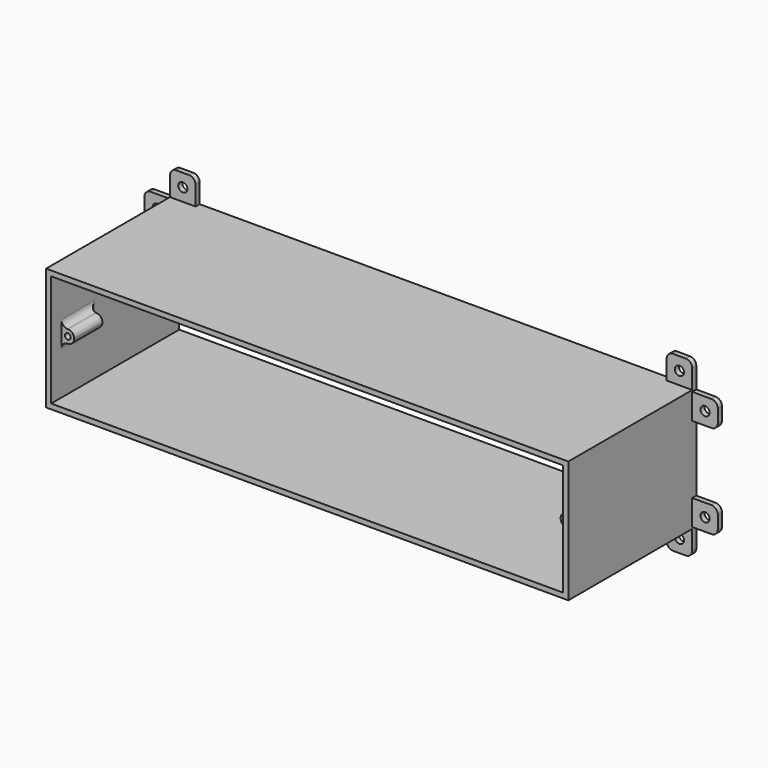
from build123d import *

# Parameters (mm, degrees)
F1_DEPTH     = 50
F0_W         = 8
F0_H         = 8
F0_R         = 1.425
F2_DEPTH     = 1.6
F3_R         = 2
F5_R         = 2
F6_START     = 35
F0_W_2       = 4
F0_H_2       = 4
F0_R_2       = 0.9
F6_DEPTH     = 11
F7_T1_DEPTH  = 11
F7_T6_DEPTH  = 4
F7_S7_R      = 0.9
F7_T8_DEPTH  = 4
F7_T13_DEPTH = 9
F7_T17_DEPTH = 16
F7_T24_DEPTH = 9
F7_T28_DEPTH = 16
F7_T31_DEPTH = 21
F9_R         = 2


# Not quite as in the source:
# - a fillet or chamfer that OpenCascade refuses, or shapes differently, is made with other operations: its cross-section is extruded or revolved along the edge and cut away or added


with BuildPart() as f1:
    # F0 (on Front) → F1 (new body)
    with BuildSketch(Plane.XZ):
        Polygon((-81.6, -18.6015841149), (-81.6, -19.1), (-73.6, -19.1), (73.6, -19.1), (81.6, -19.1), (81.6, -18.6015841149), (81.6, -10.6015841149), (81.6, 10.6015841149), (81.6, 18.6015841149), (81.6, 19.1), (73.6, 19.1), (-73.6, 19.1), (-81.6, 19.1), (-81.6, 18.6015841149), (-81.6, 10.6015841149), (-81.6, -10.6015841149), align=None)
        Polygon((80, -2), (80, -17.5), (-80, -17.5), (-80, 17.5), (80, 17.5), (80, 2), align=None, mode=Mode.SUBTRACT)
    extrude(amount=F1_DEPTH)

    # F0 (on Front) → F2 (join)
    with BuildSketch(Plane.XZ):
        Polygon((-81.6, -18.6015841149), (-81.6, -19.1), (-73.6, -19.1), (73.6, -19.1), (81.6, -19.1), (81.6, -18.6015841149), (81.6, -10.6015841149), (81.6, 10.6015841149), (81.6, 18.6015841149), (81.6, 19.1), (73.6, 19.1), (-73.6, 19.1), (-81.6, 19.1), (-81.6, 18.6015841149), (-81.6, 10.6015841149), (-81.6, -10.6015841149), align=None)
        Polygon((80, -2), (80, -17.5), (-80, -17.5), (-80, 17.5), (80, 17.5), (80, 2), align=None, mode=Mode.SUBTRACT)
        with Locations((-77.6, -23.1)):
            Rectangle(F0_W, F0_H)
        with Locations((-77.6, -23.1)):
            Circle(F0_R, mode=Mode.SUBTRACT)
        with Locations((-85.6, -14.6015841149)):
            Rectangle(F0_W, F0_H)
        with Locations((-85.6, -14.6015841149)):
            Circle(F0_R, mode=Mode.SUBTRACT)
        with Locations((77.6, -23.1)):
            Rectangle(F0_W, F0_H)
        with Locations((77.6, -23.1)):
            Circle(F0_R, mode=Mode.SUBTRACT)
        with Locations((-85.6, 14.6015841149)):
            Rectangle(F0_W, F0_H)
        with Locations((-85.6, 14.6015841149)):
            Circle(F0_R, mode=Mode.SUBTRACT)
        with Locations((85.6, -14.6015841149)):
            Rectangle(F0_W, F0_H)
        with Locations((85.6, -14.6015841149)):
            Circle(F0_R, mode=Mode.SUBTRACT)
        with Locations((-77.6, 23.1)):
            Rectangle(F0_W, F0_H)
        with Locations((-77.6, 23.1)):
            Circle(F0_R, mode=Mode.SUBTRACT)
        with Locations((85.6, 14.6015841149)):
            Rectangle(F0_W, F0_H)
        with Locations((85.6, 14.6015841149)):
            Circle(F0_R, mode=Mode.SUBTRACT)
        with Locations((77.6, 23.1)):
            Rectangle(F0_W, F0_H)
        with Locations((77.6, 23.1)):
            Circle(F0_R, mode=Mode.SUBTRACT)
    extrude(amount=F2_DEPTH)

    # F3
    f3_edges = [f1.edges().sort_by_distance(p)[0] for p in [
        (-81.6, -0.8, 27.1),
        (-73.6, -0.8, 27.1),
        (73.6, -0.8, 27.1),
        (81.6, -0.8, 27.1),
        (89.6, -0.8, -10.601584),
        (89.6, -0.8, -18.601584),
        (81.6, -0.8, -27.1),
        (73.6, -0.8, -27.1),
        (-89.6, -0.8, -18.601584),
        (-89.6, -0.8, -10.601584),
        (-81.6, -0.8, -27.1),
    ]]
    fillet(f3_edges, radius=F3_R)

    # F4: F1 across plane


with BuildPart() as f1_1:
    add(f1.part)
    add(f1.part.mirror(Plane.YZ))

    # F5
    f5_edges = [f1_1.edges().sort_by_distance(p)[0] for p in [
        (-73.6, -0.8, -27.1),
        (73.6, -0.8, -27.1),
    ]]
    fillet(f5_edges, radius=F5_R)

    # F0 (on Front) → F6 (join)
    with BuildSketch(Plane.XZ.offset(F6_START)):
        with Locations((78, 0)):
            Rectangle(F0_W_2, F0_H_2)
        with Locations((78, 0)):
            Circle(F0_R_2, mode=Mode.SUBTRACT)
    extrude(amount=F6_DEPTH)

    # F7: fillet of radius 2 on 5 edges, made by hand

    # F7_s2 → F7_t1 (join)
    with BuildSketch(Plane.XZ.offset(35)):
        with BuildLine():
            ThreePointArc((80, -4), (79.4142135624, -2.5857864376), (78, -2))
            Line((78, -2), (80, -2))
            Line((80, -2), (80, -4))
        make_face()
        with BuildLine():
            ThreePointArc((80, 4), (79.4142135624, 2.5857864376), (78, 2))
            Line((78, 2), (80, 2))
            Line((80, 2), (80, 4))
        make_face()
    extrude(amount=F7_T1_DEPTH)


with BuildPart() as f7_tool4:
    # F7_s5 → F7_t6 (new body)
    with BuildSketch(Plane.XY.offset(-2)):
        with BuildLine():
            ThreePointArc((80, -33), (79.4142135624, -34.4142135624), (78, -35))
            Line((78, -35), (80, -35))
            Line((80, -35), (80, -33))
        make_face()
    extrude(amount=F7_T6_DEPTH)

    # F7_s7 → F7_t8 (cut, symmetric)
    with BuildSketch(Plane.XZ.offset(34)):
        with Locations((78, 0)):
            Circle(F7_S7_R)
    extrude(amount=F7_T8_DEPTH, both=True, mode=Mode.SUBTRACT)


with BuildPart() as f1_2:
    add(f1_1.part)

    # F7_t3: union F7_tool4
    add(f7_tool4.part)


with BuildPart() as f7_tool11:
    # F7_s12 → F7_t13 (new body)
    with BuildSketch(Plane.XY.offset(-7)):
        with BuildLine():
            ThreePointArc((80, -33), (79.4142135624, -34.4142135624), (78, -35))
            Line((78, -35), (80, -35))
            Line((80, -35), (80, -33))
        make_face()
    extrude(amount=F7_T13_DEPTH)

    split(bisect_by=Plane.XY.offset(-2), keep=Keep.BOTTOM)


with BuildPart() as f7_tool15:
    # F7_s16 → F7_t17 (new body)
    with BuildSketch(Plane.XZ.offset(30)):
        with BuildLine():
            ThreePointArc((80, -4), (79.4142135624, -2.5857864376), (78, -2))
            Line((78, -2), (80, -2))
            Line((80, -2), (80, -4))
        make_face()
    extrude(amount=F7_T17_DEPTH)

    split(bisect_by=Plane.XZ.offset(35), keep=Keep.BOTTOM)


with BuildPart() as f7_tool11_1:
    add(f7_tool11.part)

    # F7_t19: intersect F7_tool15
    add(f7_tool15.part, mode=Mode.INTERSECT)


with BuildPart() as f1_3:
    add(f1_2.part)

    # F7_t9: union F7_tool11
    add(f7_tool11_1.part)


with BuildPart() as f7_tool22:
    # F7_s23 → F7_t24 (new body)
    with BuildSketch(Plane.XY.offset(-2)):
        with BuildLine():
            ThreePointArc((80, -33), (79.4142135624, -34.4142135624), (78, -35))
            Line((78, -35), (80, -35))
            Line((80, -35), (80, -33))
        make_face()
    extrude(amount=F7_T24_DEPTH)

    split(bisect_by=Plane.XY.offset(2), keep=Keep.TOP)


with BuildPart() as f7_tool26:
    # F7_s27 → F7_t28 (new body)
    with BuildSketch(Plane.XZ.offset(30)):
        with BuildLine():
            ThreePointArc((80, 4), (79.4142135624, 2.5857864376), (78, 2))
            Line((78, 2), (80, 2))
            Line((80, 2), (80, 4))
        make_face()
    extrude(amount=F7_T28_DEPTH)

    split(bisect_by=Plane.XZ.offset(35), keep=Keep.BOTTOM)


with BuildPart() as f7_tool22_1:
    add(f7_tool22.part)

    # F7_t30: intersect F7_tool26
    add(f7_tool26.part, mode=Mode.INTERSECT)


with BuildPart() as f1_4:
    add(f1_3.part)

    # F7_t20: union F7_tool22
    add(f7_tool22_1.part)

    # F7_s32 → F7_t31 (cut)
    with BuildSketch(Plane.XZ.offset(30)):
        with BuildLine():
            ThreePointArc((78, -2), (76.5857864376, -1.4142135624), (76, 0))
            Line((76, 0), (76, -2))
            Line((76, -2), (78, -2))
        make_face()
        with BuildLine():
            ThreePointArc((78, 2), (76.5857864376, 1.4142135624), (76, 0))
            Line((76, 0), (76, 2))
            Line((76, 2), (78, 2))
        make_face()
    extrude(amount=F7_T31_DEPTH, mode=Mode.SUBTRACT)

    # F8: F1 across plane


with BuildPart() as f1_5:
    add(f1_4.part)
    add(f1_4.part.mirror(Plane.YZ))

    # F9
    f9_edges = [f1_5.edges().sort_by_distance(p)[0] for p in [
        (89.6, -0.8, 10.601584),
        (89.6, -0.8, 18.601584),
        (-89.6, -0.8, 10.601584),
        (-89.6, -0.8, 18.601584),
    ]]
    fillet(f9_edges, radius=F9_R)


solid = f1_5.part
